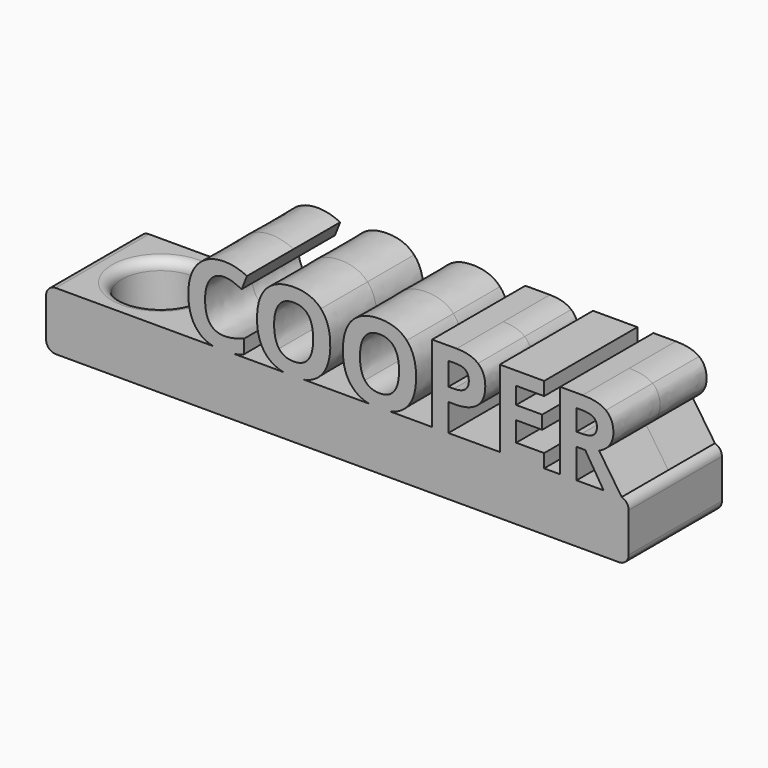
from build123d import *

# Parameters (mm, degrees)
F2_DEPTH    = 3
F3_DEPTH    = 3
F4_DEPTH    = 10
F5_T1_DEPTH = 8.5
F5_T3_DEPTH = 8.4000967976
F6_R        = 0.5
F7_R        = 0.5


# Not quite as in the source:
# - a fillet or chamfer that OpenCascade refuses, or shapes differently, is made with other operations: its cross-section is extruded or revolved along the edge and cut away or added


with BuildPart() as f2:
    # F0 (on Front) → F2 (new body)
    with BuildSketch(Plane.XZ):
        with BuildLine():
            Line((0, 3), (0, 0))
            Line((0, 0), (30, 0))
            Line((30, 0), (30, 3))
            Line((30, 3), (29.6399336075, 3))
            Line((29.6399336075, 3), (28.7072315063, 3))
            Line((28.7072315063, 3), (27.3138179486, 3))
            Line((27.3138179486, 3), (26.4730846128, 3))
            Line((26.4730846128, 3), (25.6462333547, 3))
            Line((25.6462333547, 3), (23.363499189, 3))
            Line((23.363499189, 3), (20.7172281112, 3))
            Line((20.7172281112, 3), (19.8764947754, 3))
            Line((19.8764947754, 3), (17.7098183662, 3))
            add(Edge.make_bspline(
                [(17.7098183662, 3), (17.4606461453, 2.9453393187), (17.1677543476, 2.9453393187)],
                knots=[0.6784981919, 0.6784981919, 0.6784981919, 1, 1, 1], degree=2))
            add(Edge.make_bspline(
                [(17.1677543476, 2.9453393187), (16.8748625498, 2.9453393187), (16.625690329, 3)],
                knots=[0, 0, 0, 0.3215018081, 0.3215018081, 0.3215018081], degree=2))
            Line((16.625690329, 3), (13.2901118514, 3))
            add(Edge.make_bspline(
                [(13.2901118514, 3), (13.0409396306, 2.9453393187), (12.7480478328, 2.9453393187)],
                knots=[0.6784981919, 0.6784981919, 0.6784981919, 1, 1, 1], degree=2))
            add(Edge.make_bspline(
                [(12.7480478328, 2.9453393187), (12.4551560351, 2.9453393187), (12.2059838142, 3)],
                knots=[0, 0, 0, 0.3215018081, 0.3215018081, 0.3215018081], degree=2))
            Line((12.2059838142, 3), (9.6968336244, 3))
            add(Edge.make_bspline(
                [(9.6968336244, 3), (9.4157695298, 2.9453393187), (9.1040024143, 2.9453393187)],
                knots=[0.4822306436, 0.4822306436, 0.4822306436, 1, 1, 1], degree=2))
            add(Edge.make_bspline(
                [(9.1040024143, 2.9453393187), (8.8248623099, 2.9453393187), (8.588095527, 3)],
                knots=[0, 0, 0, 0.3226952609, 0.3226952609, 0.3226952609], degree=2))
            Line((8.588095527, 3), (0, 3))
        make_face()
        with BuildLine():
            add(Edge.make_bspline(
                [(8.588095527, 3), (8.0911459788, 3.1147272457), (7.7808668754, 3.470255385)],
                knots=[0.3226952609, 0.3226952609, 0.3226952609, 1, 1, 1], degree=2))
            Line((8.588095527, 3), (9.6968336244, 3))
            add(Edge.make_bspline(
                [(10.1937455204, 3.1492323362), (9.9586060093, 3.0509088751), (9.6968336244, 3)],
                knots=[0, 0, 0, 0.4822306436, 0.4822306436, 0.4822306436], degree=2))
            Line((10.1937455204, 3.1492323362), (10.1937455204, 3.8537477838))
            add(Edge.make_bspline(
                [(9.1829567317, 3.645516617), (9.6002866951, 3.645516617), (10.1937455204, 3.8537477838)],
                knots=[0, 0, 0, 1, 1, 1], degree=2))
            add(Edge.make_bspline(
                [(8.1877852805, 4.9712550455), (8.1877852805, 3.645516617), (9.1829567317, 3.645516617)],
                knots=[0, 0, 0, 1, 1, 1], degree=2))
            add(Edge.make_bspline(
                [(8.4480742389, 5.9646912369), (8.1877852805, 5.6080953638), (8.1877852805, 4.9712550455)],
                knots=[0, 0, 0, 1, 1, 1], degree=2))
            add(Edge.make_bspline(
                [(9.1829567317, 6.32128711), (8.7083631974, 6.32128711), (8.4480742389, 5.9646912369)],
                knots=[0, 0, 0, 1, 1, 1], degree=2))
            add(Edge.make_bspline(
                [(9.6245803312, 6.2427666076), (9.3998641971, 6.32128711), (9.1829567317, 6.32128711)],
                knots=[0, 0, 0, 1, 1, 1], degree=2))
            add(Edge.make_bspline(
                [(10.0722773398, 6.058395262), (9.8492964654, 6.1642461051), (9.6245803312, 6.2427666076)],
                knots=[0, 0, 0, 1, 1, 1], degree=2))
            Line((10.0722773398, 6.058395262), (10.3429778566, 6.7420875929))
            add(Edge.make_bspline(
                [(9.1829567317, 7.0205967785), (9.7599305896, 7.0205967785), (10.3429778566, 6.7420875929)],
                knots=[0, 0, 0, 1, 1, 1], degree=2))
            add(Edge.make_bspline(
                [(8.1947263194, 6.772888453), (8.6163944321, 7.0205967785), (9.1829567317, 7.0205967785)],
                knots=[0, 0, 0, 1, 1, 1], degree=2))
            add(Edge.make_bspline(
                [(7.5479082576, 6.0601305217), (7.7730582066, 6.5251801275), (8.1947263194, 6.772888453)],
                knots=[0, 0, 0, 1, 1, 1], degree=2))
            add(Edge.make_bspline(
                [(7.3227583085, 4.9764608246), (7.3227583085, 5.5950809159), (7.5479082576, 6.0601305217)],
                knots=[0, 0, 0, 1, 1, 1], degree=2))
            add(Edge.make_bspline(
                [(7.7808668754, 3.470255385), (7.3227583085, 3.9951714512), (7.3227583085, 4.9764608246)],
                knots=[0, 0, 0, 1, 1, 1], degree=2))
        make_face()
        with BuildLine():
            Line((9.6968336244, 3), (8.588095527, 3))
            add(Edge.make_bspline(
                [(9.1040024143, 2.9453393187), (8.8248623099, 2.9453393187), (8.588095527, 3)],
                knots=[0, 0, 0, 0.3226952609, 0.3226952609, 0.3226952609], degree=2))
            add(Edge.make_bspline(
                [(9.6968336244, 3), (9.4157695298, 2.9453393187), (9.1040024143, 2.9453393187)],
                knots=[0.4822306436, 0.4822306436, 0.4822306436, 1, 1, 1], degree=2))
        make_face()
        with BuildLine():
            Line((28.7072315063, 3), (29.6399336075, 3))
            add(Edge.make_bspline(
                [(28.4738390735, 4.7274510544), (29.3692330906, 3.3904334377), (29.6399336075, 3)],
                knots=[0, 0, 0, 1, 1, 1], degree=2))
            add(Edge.make_bspline(
                [(29.0191444415, 5.1543249462), (28.8269644272, 4.8818891697), (28.4738390735, 4.7274510544)],
                knots=[0, 0, 0, 1, 1, 1], degree=2))
            add(Edge.make_bspline(
                [(29.2113244558, 5.776415557), (29.2113244558, 5.4267607228), (29.0191444415, 5.1543249462)],
                knots=[0, 0, 0, 1, 1, 1], degree=2))
            add(Edge.make_bspline(
                [(28.8239277227, 6.6700743144), (29.2113244558, 6.3759477913), (29.2113244558, 5.776415557)],
                knots=[0, 0, 0, 1, 1, 1], degree=2))
            add(Edge.make_bspline(
                [(27.6278999585, 6.9642008375), (28.4365309895, 6.9642008375), (28.8239277227, 6.6700743144)],
                knots=[0, 0, 0, 1, 1, 1], degree=2))
            Line((27.6278999585, 6.9642008375), (26.4730846128, 6.9642008375))
            Line((26.4730846128, 6.9642008375), (26.4730846128, 3))
            Line((26.4730846128, 3), (27.3138179486, 3))
            Line((27.3138179486, 3), (27.3138179486, 4.5209551473))
            Line((27.3138179486, 4.5209551473), (27.7606473273, 4.5209551473))
            Line((27.7606473273, 4.5209551473), (28.7072315063, 3))
        make_face()
        with BuildLine():
            Line((27.5845184654, 5.2046474782), (27.3138179486, 5.2046474782))
            Line((27.3138179486, 5.2046474782), (27.3138179486, 6.2753027274))
            Line((27.3138179486, 6.2753027274), (27.5689011279, 6.2753027274))
            add(Edge.make_bspline(
                [(28.1688671772, 6.1560036214), (27.9749519031, 6.2753027274), (27.5689011279, 6.2753027274)],
                knots=[0, 0, 0, 1, 1, 1], degree=2))
            add(Edge.make_bspline(
                [(28.3627824512, 5.7547248104), (28.3627824512, 6.0367045154), (28.1688671772, 6.1560036214)],
                knots=[0, 0, 0, 1, 1, 1], degree=2))
            add(Edge.make_bspline(
                [(28.1732053265, 5.337394847), (28.3627824512, 5.4701422159), (28.3627824512, 5.7547248104)],
                knots=[0, 0, 0, 1, 1, 1], degree=2))
            add(Edge.make_bspline(
                [(27.5845184654, 5.2046474782), (27.9836282017, 5.2046474782), (28.1732053265, 5.337394847)],
                knots=[0, 0, 0, 1, 1, 1], degree=2))
        make_face(mode=Mode.SUBTRACT)
        with BuildLine():
            add(Edge.make_bspline(
                [(12.2059838142, 3), (11.680130158, 3.1153560337), (11.3489946811, 3.4741597193)],
                knots=[0.3215018081, 0.3215018081, 0.3215018081, 1, 1, 1], degree=2))
            Line((12.2059838142, 3), (13.2901118514, 3))
            add(Edge.make_bspline(
                [(14.1471009846, 3.4741597193), (13.8159655077, 3.1153560337), (13.2901118514, 3)],
                knots=[0, 0, 0, 0.6784981919, 0.6784981919, 0.6784981919], degree=2))
            add(Edge.make_bspline(
                [(14.6351427817, 4.9877400128), (14.6351427817, 4.00298012), (14.1471009846, 3.4741597193)],
                knots=[0, 0, 0, 1, 1, 1], degree=2))
            add(Edge.make_bspline(
                [(14.1510053189, 6.5004526764), (14.6351427817, 5.9742351654), (14.6351427817, 4.9877400128)],
                knots=[0, 0, 0, 1, 1, 1], degree=2))
            add(Edge.make_bspline(
                [(12.753253612, 7.0266701875), (13.6668678562, 7.0266701875), (14.1510053189, 6.5004526764)],
                knots=[0, 0, 0, 1, 1, 1], degree=2))
            add(Edge.make_bspline(
                [(11.3502961258, 6.5047908258), (11.8396393678, 7.0266701875), (12.753253612, 7.0266701875)],
                knots=[0, 0, 0, 1, 1, 1], degree=2))
            add(Edge.make_bspline(
                [(10.8609528839, 4.992945792), (10.8609528839, 5.982911464), (11.3502961258, 6.5047908258)],
                knots=[0, 0, 0, 1, 1, 1], degree=2))
            add(Edge.make_bspline(
                [(11.3489946811, 3.4741597193), (10.8609528839, 4.00298012), (10.8609528839, 4.992945792)],
                knots=[0, 0, 0, 1, 1, 1], degree=2))
        make_face()
        with BuildLine():
            add(Edge.make_bspline(
                [(11.7424648233, 4.9877400128), (11.7424648233, 4.3231355389), (11.994511298, 3.9869289675)],
                knots=[0, 0, 0, 1, 1, 1], degree=2))
            add(Edge.make_bspline(
                [(11.9971141876, 5.9889848731), (11.7424648233, 5.6514768569), (11.7424648233, 4.9877400128)],
                knots=[0, 0, 0, 1, 1, 1], degree=2))
            add(Edge.make_bspline(
                [(12.753253612, 6.3264928892), (12.251763552, 6.3264928892), (11.9971141876, 5.9889848731)],
                knots=[0, 0, 0, 1, 1, 1], degree=2))
            add(Edge.make_bspline(
                [(13.7536308424, 4.9877400128), (13.7536308424, 6.3264928892), (12.753253612, 6.3264928892)],
                knots=[0, 0, 0, 1, 1, 1], degree=2))
            add(Edge.make_bspline(
                [(12.7480478328, 3.6507223962), (13.7536308424, 3.6507223962), (13.7536308424, 4.9877400128)],
                knots=[0, 0, 0, 1, 1, 1], degree=2))
            add(Edge.make_bspline(
                [(11.994511298, 3.9869289675), (12.2465577728, 3.6507223962), (12.7480478328, 3.6507223962)],
                knots=[0, 0, 0, 1, 1, 1], degree=2))
        make_face(mode=Mode.SUBTRACT)
        with BuildLine():
            Line((13.2901118514, 3), (12.2059838142, 3))
            add(Edge.make_bspline(
                [(12.7480478328, 2.9453393187), (12.4551560351, 2.9453393187), (12.2059838142, 3)],
                knots=[0, 0, 0, 0.3215018081, 0.3215018081, 0.3215018081], degree=2))
            add(Edge.make_bspline(
                [(13.2901118514, 3), (13.0409396306, 2.9453393187), (12.7480478328, 2.9453393187)],
                knots=[0.6784981919, 0.6784981919, 0.6784981919, 1, 1, 1], degree=2))
        make_face()
        with BuildLine():
            add(Edge.make_bspline(
                [(16.625690329, 3), (16.0998366727, 3.1153560337), (15.7687011958, 3.4741597193)],
                knots=[0.3215018081, 0.3215018081, 0.3215018081, 1, 1, 1], degree=2))
            Line((16.625690329, 3), (17.7098183662, 3))
            add(Edge.make_bspline(
                [(18.5668074993, 3.4741597193), (18.2356720224, 3.1153560337), (17.7098183662, 3)],
                knots=[0, 0, 0, 0.6784981919, 0.6784981919, 0.6784981919], degree=2))
            add(Edge.make_bspline(
                [(19.0548492965, 4.9877400128), (19.0548492965, 4.00298012), (18.5668074993, 3.4741597193)],
                knots=[0, 0, 0, 1, 1, 1], degree=2))
            add(Edge.make_bspline(
                [(18.5707118337, 6.5004526764), (19.0548492965, 5.9742351654), (19.0548492965, 4.9877400128)],
                knots=[0, 0, 0, 1, 1, 1], degree=2))
            add(Edge.make_bspline(
                [(17.1729601267, 7.0266701875), (18.086574371, 7.0266701875), (18.5707118337, 6.5004526764)],
                knots=[0, 0, 0, 1, 1, 1], degree=2))
            add(Edge.make_bspline(
                [(15.7700026406, 6.5047908258), (16.2593458825, 7.0266701875), (17.1729601267, 7.0266701875)],
                knots=[0, 0, 0, 1, 1, 1], degree=2))
            add(Edge.make_bspline(
                [(15.2806593987, 4.992945792), (15.2806593987, 5.982911464), (15.7700026406, 6.5047908258)],
                knots=[0, 0, 0, 1, 1, 1], degree=2))
            add(Edge.make_bspline(
                [(15.7687011958, 3.4741597193), (15.2806593987, 4.00298012), (15.2806593987, 4.992945792)],
                knots=[0, 0, 0, 1, 1, 1], degree=2))
        make_face()
        with BuildLine():
            add(Edge.make_bspline(
                [(16.162171338, 4.9877400128), (16.162171338, 4.3231355389), (16.4142178128, 3.9869289675)],
                knots=[0, 0, 0, 1, 1, 1], degree=2))
            add(Edge.make_bspline(
                [(16.4168207024, 5.9889848731), (16.162171338, 5.6514768569), (16.162171338, 4.9877400128)],
                knots=[0, 0, 0, 1, 1, 1], degree=2))
            add(Edge.make_bspline(
                [(17.1729601267, 6.3264928892), (16.6714700668, 6.3264928892), (16.4168207024, 5.9889848731)],
                knots=[0, 0, 0, 1, 1, 1], degree=2))
            add(Edge.make_bspline(
                [(18.1733373571, 4.9877400128), (18.1733373571, 6.3264928892), (17.1729601267, 6.3264928892)],
                knots=[0, 0, 0, 1, 1, 1], degree=2))
            add(Edge.make_bspline(
                [(17.1677543476, 3.6507223962), (18.1733373571, 3.6507223962), (18.1733373571, 4.9877400128)],
                knots=[0, 0, 0, 1, 1, 1], degree=2))
            add(Edge.make_bspline(
                [(16.4142178128, 3.9869289675), (16.6662642876, 3.6507223962), (17.1677543476, 3.6507223962)],
                knots=[0, 0, 0, 1, 1, 1], degree=2))
        make_face(mode=Mode.SUBTRACT)
        with BuildLine():
            Line((17.7098183662, 3), (16.625690329, 3))
            add(Edge.make_bspline(
                [(17.1677543476, 2.9453393187), (16.8748625498, 2.9453393187), (16.625690329, 3)],
                knots=[0, 0, 0, 0.3215018081, 0.3215018081, 0.3215018081], degree=2))
            add(Edge.make_bspline(
                [(17.7098183662, 3), (17.4606461453, 2.9453393187), (17.1677543476, 2.9453393187)],
                knots=[0.6784981919, 0.6784981919, 0.6784981919, 1, 1, 1], degree=2))
        make_face()
        Polygon((23.363499189, 3), (25.6462333547, 3), (25.6462333547, 3.6941038892), (24.2042325248, 3.6941038892), (24.2042325248, 4.7161718662), (25.5464559206, 4.7161718662), (25.5464559206, 5.4050699762), (24.2042325248, 5.4050699762), (24.2042325248, 6.2753027274), (25.6462333547, 6.2753027274), (25.6462333547, 6.9642008375), (23.363499189, 6.9642008375), align=None)
        with BuildLine():
            Line((19.8764947754, 6.9642008375), (19.8764947754, 3))
            Line((19.8764947754, 3), (20.7172281112, 3))
            Line((20.7172281112, 3), (20.7172281112, 4.409898525))
            Line((20.7172281112, 4.409898525), (21.0772945038, 4.409898525))
            add(Edge.make_bspline(
                [(22.2147572523, 4.748707986), (21.8147798861, 4.409898525), (21.0772945038, 4.409898525)],
                knots=[0, 0, 0, 1, 1, 1], degree=2))
            add(Edge.make_bspline(
                [(22.6147346184, 5.7278282847), (22.6147346184, 5.0875174469), (22.2147572523, 4.748707986)],
                knots=[0, 0, 0, 1, 1, 1], degree=2))
            add(Edge.make_bspline(
                [(22.2394847033, 6.653589347), (22.6147346184, 6.3429778566), (22.6147346184, 5.7278282847)],
                knots=[0, 0, 0, 1, 1, 1], degree=2))
            add(Edge.make_bspline(
                [(21.1423667434, 6.9642008375), (21.8642347882, 6.9642008375), (22.2394847033, 6.653589347)],
                knots=[0, 0, 0, 1, 1, 1], degree=2))
            Line((21.1423667434, 6.9642008375), (19.8764947754, 6.9642008375))
        make_face()
        with BuildLine():
            Line((20.994002037, 5.0987966351), (20.7172281112, 5.0987966351))
            Line((20.7172281112, 5.0987966351), (20.7172281112, 6.2753027274))
            Line((20.7172281112, 6.2753027274), (21.0989852503, 6.2753027274))
            add(Edge.make_bspline(
                [(21.6048134596, 6.1343128749), (21.4434343053, 6.2753027274), (21.0989852503, 6.2753027274)],
                knots=[0, 0, 0, 1, 1, 1], degree=2))
            add(Edge.make_bspline(
                [(21.7661926138, 5.6974612396), (21.7661926138, 5.9933230224), (21.6048134596, 6.1343128749)],
                knots=[0, 0, 0, 1, 1, 1], degree=2))
            add(Edge.make_bspline(
                [(21.5735787846, 5.2519333057), (21.7661926138, 5.4050699762), (21.7661926138, 5.6974612396)],
                knots=[0, 0, 0, 1, 1, 1], degree=2))
            add(Edge.make_bspline(
                [(20.994002037, 5.0987966351), (21.3809649553, 5.0987966351), (21.5735787846, 5.2519333057)],
                knots=[0, 0, 0, 1, 1, 1], degree=2))
        make_face(mode=Mode.SUBTRACT)
    extrude(amount=F2_DEPTH)

    # F3 (add): a face of the model
    f3_faces = [f2.faces().sort_by_distance(p)[0] for p in [
        (16.1900363692, 0, 2.6380642598),
    ]]
    extrude(f3_faces, amount=F3_DEPTH)

    # F1 (on Top) → F4 (cut)
    with BuildSketch(Plane.XY):
        with BuildLine():
            ThreePointArc((1.5, 0), (3.5, -2), (5.5, 0))
            ThreePointArc((5.5, 0), (3.5, 2), (1.5, 0))
        make_face()
    extrude(amount=F4_DEPTH, mode=Mode.SUBTRACT)

    # F5: fillet of radius 0.5 on 2 edges, made by hand

    # F5_s2 → F5_t1 (cut)
    with BuildSketch(Plane.XZ.offset(-4.25)):
        with BuildLine():
            ThreePointArc((29.5, 0), (29.8535533906, 0.1464466094), (30, 0.5))
            Line((30, 0.5), (30.01, 0.5))
            Line((30.01, 0.5), (30.01, -0.01))
            Line((30.01, -0.01), (29.5, -0.01))
            Line((29.5, -0.01), (29.5, 0))
        make_face()
    extrude(amount=F5_T1_DEPTH, mode=Mode.SUBTRACT)

    # F5_s4 → F5_t3 (cut)
    with BuildSketch(Plane.XZ.offset(-4.2000483988)):
        with BuildLine():
            ThreePointArc((30, 2.5199806405), (29.8999792518, 2.8200083028), (29.6399336075, 3))
            Line((29.6399336075, 3), (29.6427322796, 3.0096003872))
            ThreePointArc((29.6427322796, 3.0096003872), (29.8199668037, 3.01), (30, 3.01))
            Line((30, 3.01), (30.01, 3))
            Line((30.01, 3), (30.01, 2.5199806405))
            Line((30.01, 2.5199806405), (30, 2.5199806405))
        make_face()
    extrude(amount=F5_T3_DEPTH, mode=Mode.SUBTRACT)

    # F6
    f6_edges = [f2.edges().sort_by_distance(p)[0] for p in [
        (0, 0, 3),
        (0, 0, 0),
    ]]
    fillet(f6_edges, radius=F6_R)

    # F7
    f7_edges = [f2.edges().sort_by_distance(p)[0] for p in [
        (1.5, 0, 3),
        (1.5, 0, 0),
    ]]
    fillet(f7_edges, radius=F7_R)


solid = f2.part
